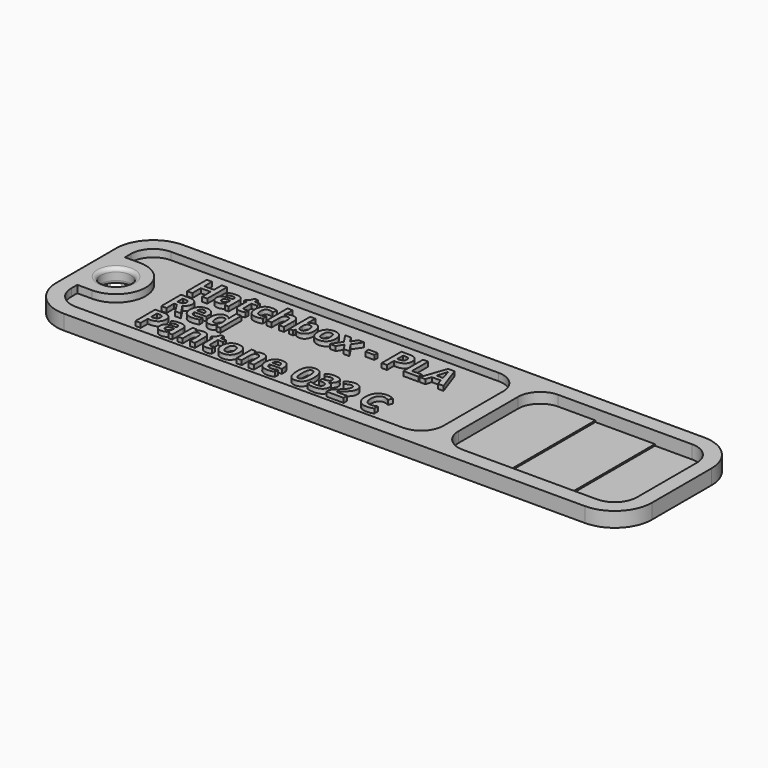
from build123d import *

# Parameters (mm, degrees)
F1_DEPTH      = 2
F3_DEPTH      = 1
F4_R          = 2
F5_DEPTH      = 2.001
F6_R          = 0.5
F7_DEPTH      = 0.4
F9_DEPTH      = 0.2
F11_DEPTH     = 0.2
F12_TEXT_SIZE = 4.6296296296
F13_DEPTH     = 0.6


# Not quite as in the source:
# - Text() gives the source's letters only with a copy of the font that has no kerning and outlines rounded to 1/6400 em; it was checked with that copy


with BuildPart() as f1:
    # F0 (on Top) → F1 (new body)
    with BuildSketch(Plane.XY):
        with BuildLine():
            ThreePointArc((40, 5), (38.5355339059, 8.5355339059), (35, 10))
            Line((35, 10), (-35, 10))
            ThreePointArc((-35, 10), (-38.5355339059, 8.5355339059), (-40, 5))
            Line((-40, 5), (-40, -5))
            ThreePointArc((-40, -5), (-38.5355339059, -8.5355339059), (-35, -10))
            Line((-35, -10), (35, -10))
            ThreePointArc((35, -10), (38.5355339059, -8.5355339059), (40, -5))
            Line((40, -5), (40, 5))
        make_face()
    extrude(amount=F1_DEPTH)

    # F2 (on face) → F3 (cut)
    with BuildSketch(Plane.XY.offset(2)):
        with BuildLine():
            ThreePointArc((35, -8), (37.1213203436, -7.1213203436), (38, -5))
            Line((38, -5), (38, 5))
            ThreePointArc((38, 5), (37.1213203436, 7.1213203436), (35, 8))
            Line((35, 8), (17, 8))
            ThreePointArc((17, 8), (14.8786796564, 7.1213203436), (14, 5))
            Line((14, 5), (14, -5))
            ThreePointArc((14, -5), (14.8786796564, -7.1213203436), (17, -8))
            Line((17, -8), (35, -8))
        make_face()
        with BuildLine():
            ThreePointArc((-38, -5), (-37.1213203436, -7.1213203436), (-35, -8))
            Line((-35, -8), (9, -8))
            ThreePointArc((9, -8), (11.1213203436, -7.1213203436), (12, -5))
            Line((12, -5), (12, 5))
            ThreePointArc((12, 5), (11.1213203436, 7.1213203436), (9, 8))
            Line((9, 8), (-35, 8))
            ThreePointArc((-35, 8), (-37.1213203436, 7.1213203436), (-38, 5))
            Line((-38, 5), (-38, 4))
            Line((-38, 4), (-36, 4))
            ThreePointArc((-36, 4), (-32, 0), (-36, -4))
            Line((-36, -4), (-38, -4))
            Line((-38, -4), (-38, -5))
        make_face()
    extrude(amount=-F3_DEPTH, mode=Mode.SUBTRACT)

    # F4 (on face) → F5 (cut, through all)
    with BuildSketch(Plane.XY.offset(2)):
        with Locations((-36, 0)):
            Circle(F4_R)
    extrude(amount=-F5_DEPTH, mode=Mode.SUBTRACT)

    # F6
    f6_edges = [f1.edges().sort_by_distance(p)[0] for p in [
        (-38, 0, 2),
        (-38, 0, 0),
    ]]
    fillet(f6_edges, radius=F6_R)

    # F7 (cut): a face of the model
    f7_faces = [f1.faces().sort_by_distance(p)[0] for p in [
        (26, 0, 1),
    ]]
    extrude(f7_faces, amount=-F7_DEPTH, mode=Mode.SUBTRACT)

    # F8 (on face) → F9 (cut)
    with BuildSketch(Plane.XY.offset(0.6)):
        with BuildLine():
            Line((22, -8), (35, -8))
            ThreePointArc((35, -8), (37.1213203436, -7.1213203436), (38, -5))
            Line((38, -5), (38, 5))
            ThreePointArc((38, 5), (37.1213203436, 7.1213203436), (35, 8))
            Line((35, 8), (22, 8))
            Line((22, 8), (22, -8))
        make_face()
    extrude(amount=-F9_DEPTH, mode=Mode.SUBTRACT)

    # F10 (on face) → F11 (cut)
    with BuildSketch(Plane.XY.offset(0.4)):
        with BuildLine():
            ThreePointArc((38, 5), (37.1213203436, 7.1213203436), (35, 8))
            Line((35, 8), (30, 8))
            Line((30, 8), (30, -8))
            Line((30, -8), (35, -8))
            ThreePointArc((35, -8), (37.1213203436, -7.1213203436), (38, -5))
            Line((38, -5), (38, 5))
        make_face()
    extrude(amount=-F11_DEPTH, mode=Mode.SUBTRACT)

    # F12 (on face) → F13 (join)
    with BuildSketch(Plane.XY.offset(1)):
        with Locations((-29, 2.6666666667)):
            Text('Hatchbox - PLA', F12_TEXT_SIZE, font='Open Sans', font_style=FontStyle.BOLD, text_align=(TextAlign.LEFT, TextAlign.BOTTOM))
        with Locations((-29, -1.6666666667)):
            Text('Red', F12_TEXT_SIZE, font='Open Sans', font_style=FontStyle.BOLD, text_align=(TextAlign.LEFT, TextAlign.BOTTOM))
        with Locations((-29, -6)):
            Text('Pantone 032 C', F12_TEXT_SIZE, font='Open Sans', font_style=FontStyle.BOLD, text_align=(TextAlign.LEFT, TextAlign.BOTTOM))
    extrude(amount=F13_DEPTH)


solid = f1.part
